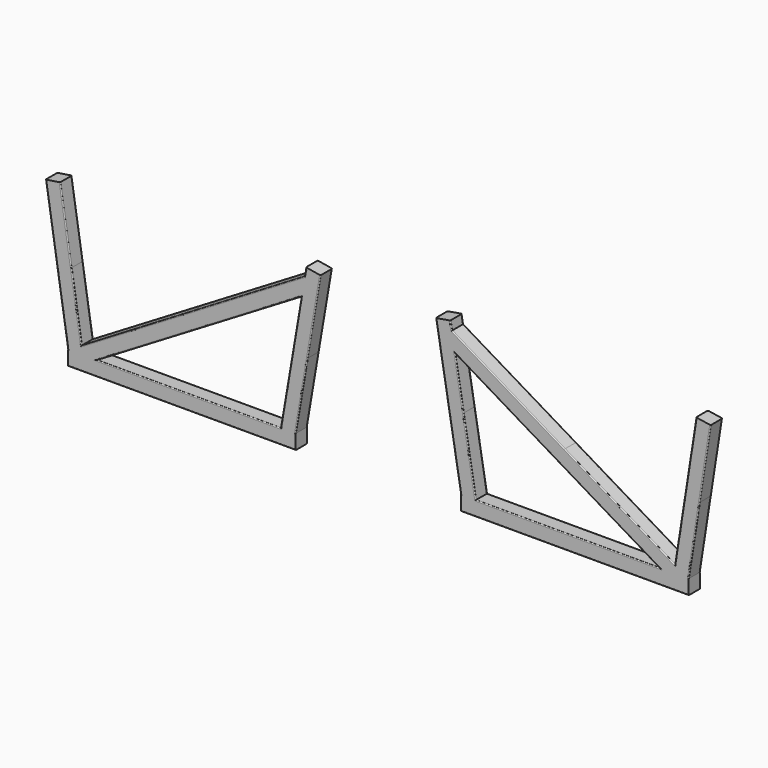
from build123d import *


with BuildPart() as f11:
    # F11: sweep along a path in F0
    with BuildLine(Plane.XZ) as f11_path:
        Line((-562.398102, -405.876424), (-543.076471, -529.856885))
        Line((-543.076471, -529.856885), (-523.7217, -654.05))
        Line((-523.7217, -654.05), (-521.742479, -666.75))
    # F7 (on line) → F11 (sweep)
    with BuildSketch(Plane(origin=(67.739956, 0, -434.664715), x_dir=(0.988073, 0, 0.153985), z_dir=(0.153985, 0, -0.988073))):
        with BuildLine():
            Line((-629.301999, -12.7), (-607.076999, -12.7))
            ThreePointArc((-607.076999, -12.7), (-605.954467, -12.235032), (-605.489499, -11.1125))
            Line((-605.489499, -11.1125), (-605.489499, 11.1125))
            ThreePointArc((-605.489499, 11.1125), (-605.954467, 12.235032), (-607.076999, 12.7))
            Line((-607.076999, 12.7), (-629.301999, 12.7))
            ThreePointArc((-629.301999, 12.7), (-630.424531, 12.235032), (-630.889499, 11.1125))
            Line((-630.889499, 11.1125), (-630.889499, -11.1125))
            ThreePointArc((-630.889499, -11.1125), (-630.424531, -12.235032), (-629.301999, -12.7))
        make_face()
    sweep(path=f11_path.line)

    # F12: sweep along a path in F0
    with BuildLine(Plane.XZ) as f12_path:
        Line((-536.575, -666.75), (-142.875, -666.75))
    # F10 (on line) → F12 (sweep)
    with BuildSketch(Plane.YZ.offset(-339.725)):
        with BuildLine():
            ThreePointArc((-12.7, -677.8625), (-12.235032, -678.985032), (-11.1125, -679.45))
            Line((-11.1125, -679.45), (11.1125, -679.45))
            ThreePointArc((11.1125, -679.45), (12.235032, -678.985032), (12.7, -677.8625))
            Line((12.7, -677.8625), (12.7, -655.6375))
            ThreePointArc((12.7, -655.6375), (12.235032, -654.514968), (11.1125, -654.05))
            Line((11.1125, -654.05), (-11.1125, -654.05))
            ThreePointArc((-11.1125, -654.05), (-12.235032, -654.514968), (-12.7, -655.6375))
            Line((-12.7, -655.6375), (-12.7, -677.8625))
        make_face()
    sweep(path=f12_path.line)

    # F13: sweep along a path in F0
    with BuildLine(Plane.XZ) as f13_path:
        Line((-120.740297, -420.520893), (-315.763429, -537.260952))
        Line((-315.763429, -537.260952), (-510.8684, -654.05))
        Line((-510.8684, -654.05), (-521.765305, -660.572843))
    # F9 (on line) → F13 (sweep)
    with BuildSketch(Plane(origin=(-469.231855, 0, -280.880293), x_dir=(0, -1, 0), z_dir=(-0.858024, 0, -0.51361))):
        with BuildLine():
            ThreePointArc((-12.7, -309.916115), (-12.235032, -311.038647), (-11.1125, -311.503615))
            Line((-11.1125, -311.503615), (11.1125, -311.503615))
            ThreePointArc((11.1125, -311.503615), (12.235032, -311.038647), (12.7, -309.916115))
            Line((12.7, -309.916115), (12.7, -287.691115))
            ThreePointArc((12.7, -287.691115), (12.235032, -286.568583), (11.1125, -286.103615))
            Line((11.1125, -286.103615), (-11.1125, -286.103615))
            ThreePointArc((-11.1125, -286.103615), (-12.235032, -286.568583), (-12.7, -287.691115))
            Line((-12.7, -287.691115), (-12.7, -309.916115))
        make_face()
    sweep(path=f13_path.line)

    # F14: sweep along a path in F0
    with BuildLine(Plane.XZ) as f14_path:
        Line((-157.909874, -666.75), (-134.848126, -530.750868))
        Line((-134.848126, -530.750868), (-112.176737, -397.053748))
    # F8 (on line) → F14 (sweep)
    with BuildSketch(Plane(origin=(-91.254421, 0, -538.143173), x_dir=(0.985925, 0, -0.167186), z_dir=(-0.167186, 0, -0.985925))):
        with BuildLine():
            Line((-55.328529, -12.7), (-33.103529, -12.7))
            ThreePointArc((-33.103529, -12.7), (-31.980997, -12.235032), (-31.516029, -11.1125))
            Line((-31.516029, -11.1125), (-31.516029, 11.1125))
            ThreePointArc((-31.516029, 11.1125), (-31.980997, 12.235032), (-33.103529, 12.7))
            Line((-33.103529, 12.7), (-55.328529, 12.7))
            ThreePointArc((-55.328529, 12.7), (-56.451061, 12.235032), (-56.916029, 11.1125))
            Line((-56.916029, 11.1125), (-56.916029, -11.1125))
            ThreePointArc((-56.916029, -11.1125), (-56.451061, -12.235032), (-55.328529, -12.7))
        make_face()
    sweep(path=f14_path.line)


with BuildPart() as f15_1:
    # F15: instance of F11
    add(f11.part.mirror(Plane.YZ))


solid = Compound([f11.part, f15_1.part])
